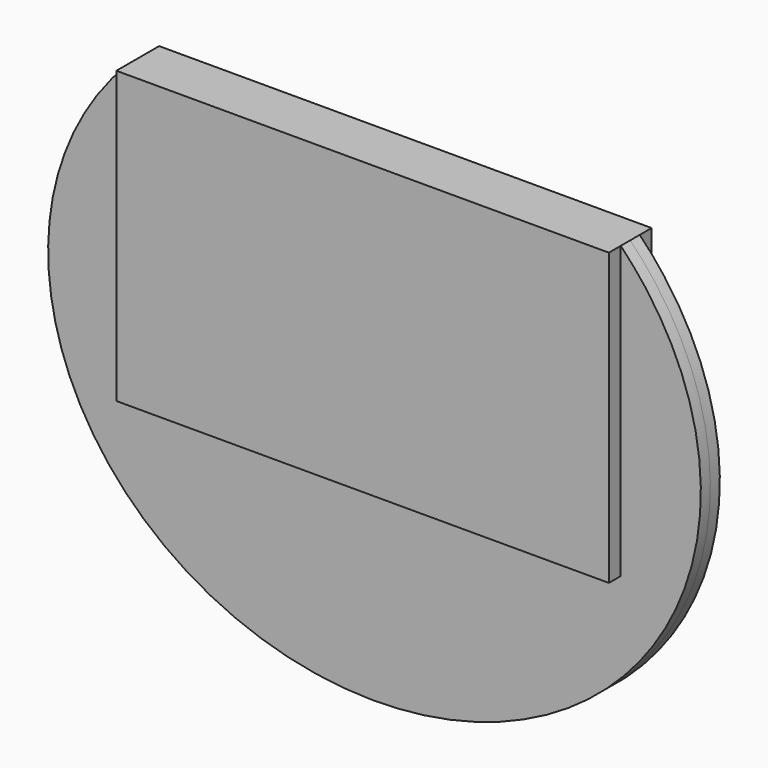
from build123d import *

# Parameters (mm, degrees)
F1_W     = 41.5
F1_H     = 24.5
F2_DEPTH = 2.25
F3_DEPTH = 1


with BuildPart() as f2:
    # F1 (on Front) → F2 (new body, symmetric)
    with BuildSketch(Plane.XZ):
        Rectangle(F1_W, F1_H)
    extrude(amount=F2_DEPTH, both=True)


with BuildPart() as f3:
    # F1 (on Front) → F3 (new body, symmetric)
    with BuildSketch(Plane.XZ):
        with BuildLine():
            Line((-20.75, -12.25), (-20.75, 12.25))
            add(Edge.make_bspline(
                [(-20.75, 12.25), (-60.3632476333, -28.25), (0, -28.25), (60.3632476333, -28.25), (20.75, 12.25)],
                knots=[2.4257575272, 2.4257575272, 2.4257575272, 4.7123889804, 4.7123889804, 6.9990204336, 6.9990204336, 6.9990204336], degree=2, weights=[1, 0.4145794337, 1, 0.4145794337, 1]))
            Line((20.75, 12.25), (20.75, -12.25))
            Line((20.75, -12.25), (-20.75, -12.25))
        make_face()
    extrude(amount=F3_DEPTH, both=True)


solid = Compound([f2.part, f3.part])
